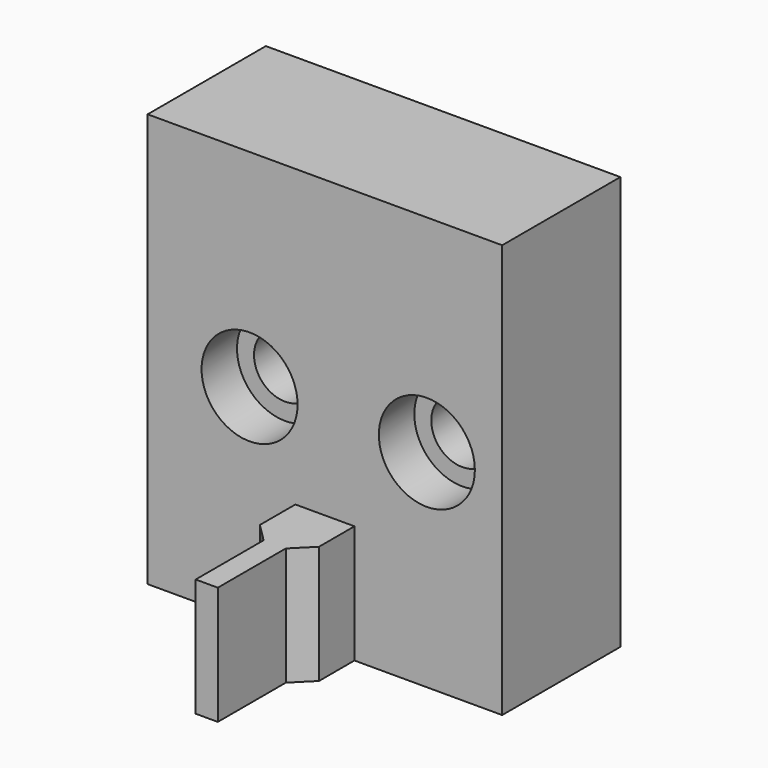
from build123d import *

# Parameters (mm, degrees)
F0_W        = 24
F0_H        = 28
F0_R        = 2.1
F1_DEPTH    = 10
F2_W        = 4
F2_H        = 8
F3_DEPTH    = 5
F4_W        = 1.5
F4_H        = 8
F5_DEPTH    = 5
F6_T4_DEPTH = 18.2867319519
F6_T9_DEPTH = 18.2867319519
F7_R        = 3.25
F8_DEPTH    = 3


# Not quite as in the source:
# - a fillet or chamfer that OpenCascade refuses, or shapes differently, is made with other operations: its cross-section is extruded or revolved along the edge and cut away or added


with BuildPart() as f1:
    # F0 (on Front) → F1 (new body)
    with BuildSketch(Plane.XZ):
        Rectangle(F0_W, F0_H)
        with Locations((-5.1, 0)):
            Circle(F0_R, mode=Mode.SUBTRACT)
        with Locations((6.9, 0)):
            Circle(F0_R, mode=Mode.SUBTRACT)
    extrude(amount=F1_DEPTH)

    # F2 (on face) → F3 (join)
    with BuildSketch(Plane.XZ.offset(10)):
        with Locations((0, -10)):
            Rectangle(F2_W, F2_H)
    extrude(amount=F3_DEPTH)

    # F4 (on face) → F5 (join)
    with BuildSketch(Plane.XZ.offset(15)):
        with Locations((0, -10)):
            Rectangle(F4_W, F4_H)
    extrude(amount=F5_DEPTH)

    # F6: chamfer of 2 on 2 edges, made by hand


with BuildPart() as f6_tool2:
    # F6_s3 → F6_t4 (new body)
    with BuildSketch(Plane.XY.offset(-19.1433659759)):
        Polygon((0, -15), (2, -13), (2, -15), align=None)
    extrude(amount=F6_T4_DEPTH)

    split(bisect_by=Plane.YZ.offset(0.75), keep=Keep.TOP)


with BuildPart() as f1_1:
    add(f1.part)

    # F6_t1: cut F6_tool2
    add(f6_tool2.part, mode=Mode.SUBTRACT)


with BuildPart() as f6_tool7:
    # F6_s8 → F6_t9 (new body)
    with BuildSketch(Plane.XY.offset(-0.8566340241)):
        Polygon((-2, -13), (0, -15), (-2, -15), align=None)
    extrude(amount=-F6_T9_DEPTH)

    split(bisect_by=Plane.YZ.offset(-0.75), keep=Keep.BOTTOM)


with BuildPart() as f1_2:
    add(f1_1.part)

    # F6_t6: cut F6_tool7
    add(f6_tool7.part, mode=Mode.SUBTRACT)

    # F7 (on face) → F8 (cut)
    with BuildSketch(Plane.XZ.offset(10)):
        with Locations((-5.1, 0)):
            Circle(F7_R)
        with Locations((6.9, 0)):
            Circle(F7_R)
    extrude(amount=-F8_DEPTH, mode=Mode.SUBTRACT)


solid = f1_2.part
